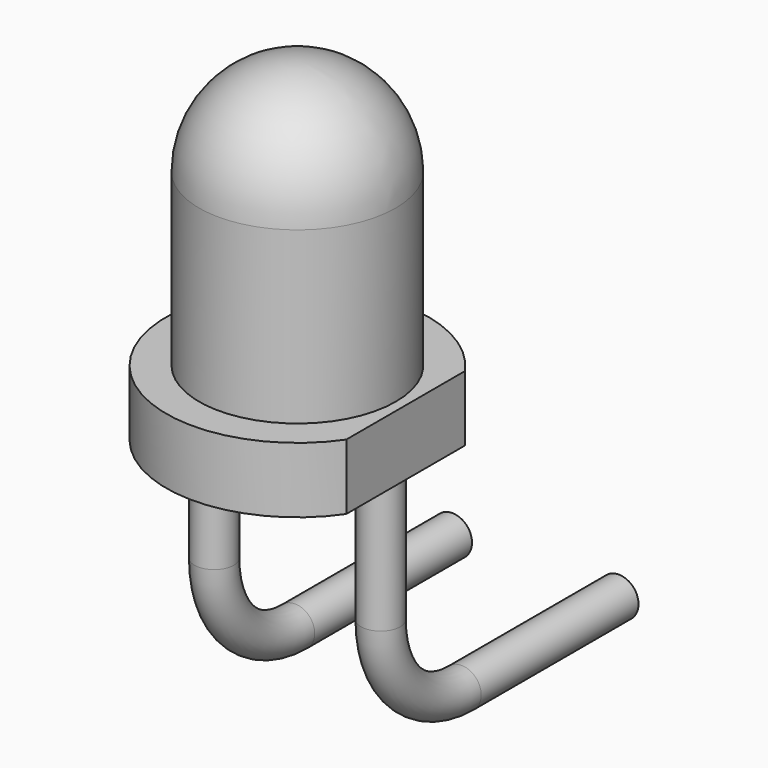
from build123d import *

# Parameters (mm, degrees)
F2_R      = 0.3
F3_DEPTH  = 2
F4_DEPTH  = 25
F5_R      = 0.3
F6_ANGLE  = 90
F6_FACE_R = 0.3
F7_R      = 0.3
F8_DEPTH  = 3


# Not quite as in the source:
# - a feature names something its author has since deleted; it is built from what else it names


with BuildPart() as f1:
    # F0 (on Front) → F1 (revolve)
    with BuildSketch(Plane.XZ):
        with BuildLine():
            Line((0, 3.6), (0, 0))
            Line((0, 0), (1.5, 0))
            Line((1.5, 0), (2, 0))
            Line((2, 0), (2, 1))
            Line((2, 1), (1.5, 1))
            Line((1.5, 1), (1.5, 3.6))
            ThreePointArc((1.5, 3.6), (1.0606601718, 4.6606601718), (0, 5.1))
            Line((0, 5.1), (0, 3.6))
        make_face()
    revolve(axis=Axis((0, 0, 1.8), (0, 0, 1)))

    # F2 (on Top) → F3 (join)
    with BuildSketch(Plane.XY):
        with Locations((-1.27, 0)):
            Circle(F2_R)
        with Locations((1.27, 0)):
            Circle(F2_R)
    extrude(amount=-F3_DEPTH)

    # F2 (on Top) → F4 (cut)
    with BuildSketch(Plane.XY):
        with BuildLine():
            Line((1.65, 1.1302654555), (1.65, 0))
            Line((1.65, 0), (1.65, -1.1302654555))
            ThreePointArc((1.65, -1.1302654555), (1.9104973175, -0.5916079783), (2, 0))
            ThreePointArc((2, 0), (1.9104973175, 0.5916079783), (1.65, 1.1302654555))
        make_face()
    extrude(amount=F4_DEPTH, mode=Mode.SUBTRACT)

    # F5 (on face) → F6 (revolve)
    with BuildSketch(Plane(origin=(0, 0, -2), x_dir=(1, 0, 0), z_dir=(0, 0, -1))):
        with Locations((-1.27, 0)):
            Circle(F5_R)
        with Locations((1.27, 0)):
            Circle(F5_R)
    revolve(axis=Axis((0.0564431539, 1.5424509184, -2), (1, 0, 0)), revolution_arc=F6_ANGLE)

    # F6_face (on face) + F7 (on face) → F8 (join)
    with BuildSketch(Plane(origin=(1.27, 1.5424509184, -3.5424509184), x_dir=(-1, 0, 0), z_dir=(0, 1, 0))):
        with Locations((2.54, 0)):
            Circle(F6_FACE_R)
    with BuildSketch(Plane(origin=(0, 1.5424509184, 0), x_dir=(-1, 0, 0), z_dir=(0, 1, 0))):
        with Locations((-1.27, -3.5424509184)):
            Circle(F7_R)
    extrude(amount=F8_DEPTH)


solid = f1.part
